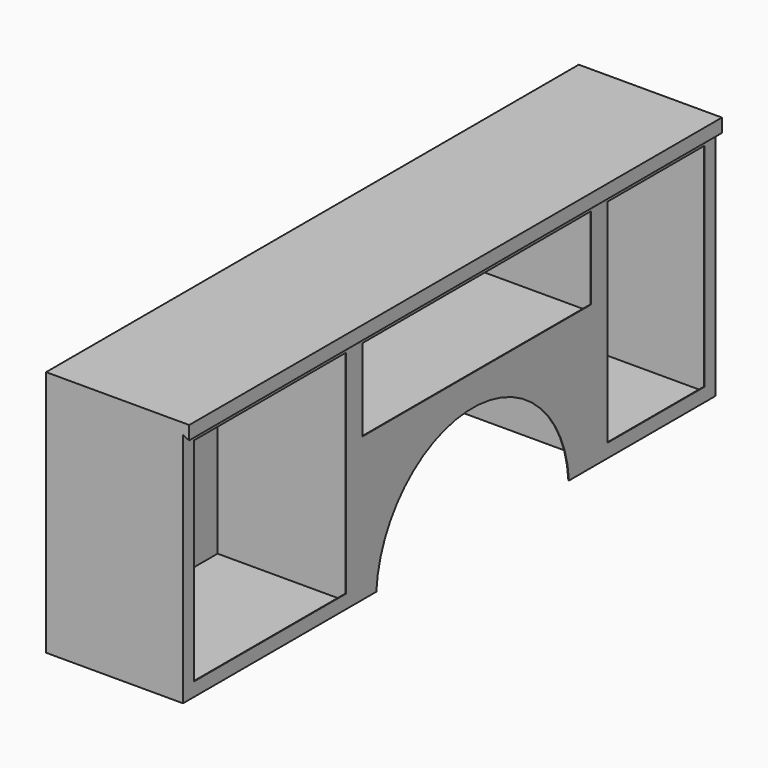
from build123d import *

# Parameters (mm, degrees)
F0_W      = 508
F0_H      = 914.4
F1_DEPTH  = 2470.15
F2_W      = 704.85
F2_H      = 787.4
F2_W_2    = 1060.45
F2_H_2    = 304.8
F2_W_3    = 450.85
F3_DEPTH  = 505.8918
F4_W      = 503.7836
F4_H      = 704.85
F5_DEPTH  = 48.6918
F6_W      = 503.7836
F6_H      = 704.85
F7_DEPTH  = 48.6918
F8_W      = 503.7836
F8_H      = 884.7836
F9_DEPTH  = 48.6918
F10_W     = 503.7836
F10_H     = 884.7836
F11_DEPTH = 37.0459
F12_W     = 503.7836
F12_H     = 1060.45
F13_DEPTH = 48.6918
F14_W     = 503.7836
F14_H     = 1060.45
F15_DEPTH = 48.6918
F16_W     = 503.7836
F16_H     = 402.1836
F17_DEPTH = 37.0459
F18_W     = 503.7836
F18_H     = 402.1836
F19_DEPTH = 37.0459
F20_W     = 503.7836
F20_H     = 450.85
F21_DEPTH = 48.6918
F22_W     = 503.7836
F22_H     = 450.85
F23_DEPTH = 48.6918
F24_W     = 503.7836
F24_H     = 884.7836
F25_DEPTH = 37.0459
F26_W     = 503.7836
F26_H     = 884.7836
F27_DEPTH = 48.6918
F28_W     = 505.8918
F28_H     = 1134.5418
F29_DEPTH = 482.6
F31_DEPTH = 508.001
F33_DEPTH = 2470.15
F34_R     = 0.508


with BuildPart() as f1:
    # F0 (on Front) → F1 (new body)
    with BuildSketch(Plane.XZ):
        Rectangle(F0_W, F0_H)
    extrude(amount=-F1_DEPTH)

    # F2 (on face) → F3 (cut)
    with BuildSketch(Plane.YZ.offset(254)):
        with Locations((403.225, -12.7)):
            Rectangle(F2_W, F2_H)
        with Locations((1362.075, 228.6)):
            Rectangle(F2_W_2, F2_H_2)
        with Locations((2193.925, -12.7)):
            Rectangle(F2_W_3, F2_H)
    extrude(amount=-F3_DEPTH, mode=Mode.SUBTRACT)

    # F4 (on face) → F5 (cut)
    with BuildSketch(Plane.XY.offset(-406.4)):
        with Locations((0, 403.225)):
            Rectangle(F4_W, F4_H)
    extrude(amount=-F5_DEPTH, mode=Mode.SUBTRACT)

    # F6 (on face) → F7 (cut)
    with BuildSketch(Plane(origin=(0, 0, 381), x_dir=(1, 0, 0), z_dir=(0, 0, -1))):
        with Locations((0, -403.225)):
            Rectangle(F6_W, F6_H)
    extrude(amount=-F7_DEPTH, mode=Mode.SUBTRACT)

    # F8 (on face) → F9 (cut)
    with BuildSketch(Plane(origin=(0, 50.8, 0), x_dir=(-1, 0, 0), z_dir=(0, 1, 0))):
        with Locations((0, -12.7)):
            Rectangle(F8_W, F8_H)
    extrude(amount=-F9_DEPTH, mode=Mode.SUBTRACT)

    # F10 (on face) → F11 (cut)
    with BuildSketch(Plane.XZ.offset(-755.65)):
        with Locations((0, -12.7)):
            Rectangle(F10_W, F10_H)
    extrude(amount=-F11_DEPTH, mode=Mode.SUBTRACT)

    # F12 (on face) → F13 (cut)
    with BuildSketch(Plane.XY.offset(76.2)):
        with Locations((0, 1362.075)):
            Rectangle(F12_W, F12_H)
    extrude(amount=-F13_DEPTH, mode=Mode.SUBTRACT)

    # F14 (on face) → F15 (cut)
    with BuildSketch(Plane(origin=(0, 0, 381), x_dir=(1, 0, 0), z_dir=(0, 0, -1))):
        with Locations((0, -1362.075)):
            Rectangle(F14_W, F14_H)
    extrude(amount=-F15_DEPTH, mode=Mode.SUBTRACT)

    # F16 (on face) → F17 (cut)
    with BuildSketch(Plane(origin=(0, 831.85, 0), x_dir=(-1, 0, 0), z_dir=(0, 1, 0))):
        with Locations((0, 228.6)):
            Rectangle(F16_W, F16_H)
    extrude(amount=-F17_DEPTH, mode=Mode.SUBTRACT)

    # F18 (on face) → F19 (cut)
    with BuildSketch(Plane.XZ.offset(-1892.3)):
        with Locations((0, 228.6)):
            Rectangle(F18_W, F18_H)
    extrude(amount=-F19_DEPTH, mode=Mode.SUBTRACT)

    # F20 (on face) → F21 (cut)
    with BuildSketch(Plane.XY.offset(-406.4)):
        with Locations((0, 2193.925)):
            Rectangle(F20_W, F20_H)
    extrude(amount=-F21_DEPTH, mode=Mode.SUBTRACT)

    # F22 (on face) → F23 (cut)
    with BuildSketch(Plane(origin=(0, 0, 381), x_dir=(1, 0, 0), z_dir=(0, 0, -1))):
        with Locations((0, -2193.925)):
            Rectangle(F22_W, F22_H)
    extrude(amount=-F23_DEPTH, mode=Mode.SUBTRACT)

    # F24 (on face) → F25 (cut)
    with BuildSketch(Plane(origin=(0, 1968.5, 0), x_dir=(-1, 0, 0), z_dir=(0, 1, 0))):
        with Locations((0, -12.7)):
            Rectangle(F24_W, F24_H)
    extrude(amount=-F25_DEPTH, mode=Mode.SUBTRACT)

    # F26 (on face) → F27 (cut)
    with BuildSketch(Plane.XZ.offset(-2419.35)):
        with Locations((0, -12.7)):
            Rectangle(F26_W, F26_H)
    extrude(amount=-F27_DEPTH, mode=Mode.SUBTRACT)

    # F28 (on face) → F29 (cut)
    with BuildSketch(Plane(origin=(0, 0, -457.2), x_dir=(1, 0, 0), z_dir=(0, 0, -1))):
        with Locations((-1.0541, -1362.075)):
            Rectangle(F28_W, F28_H)
    extrude(amount=-F29_DEPTH, mode=Mode.SUBTRACT)

    # F30 (on face) → F31 (cut, through all)
    with BuildSketch(Plane.YZ.offset(254)):
        with BuildLine():
            Line((896.4041, -457.2), (1789.6459, -457.2))
            ThreePointArc((1789.6459, -457.2), (1343.025, -38.1), (896.4041, -457.2))
        make_face()
    extrude(amount=-F31_DEPTH, mode=Mode.SUBTRACT)

    # F32 (on face) → F33 (join, through all)
    with BuildSketch(Plane.XZ):
        Polygon((277.0862247403, 459.3082), (-254, 459.3082), (-254, 457.2), (254, 457.2), (254, 419.1), (277.0862247403, 408.5082), align=None)
    extrude(amount=-F33_DEPTH)

    # F34
    f34_edges = [f1.edges().sort_by_distance(p)[0] for p in [
        (277.086225, 1235.075, 408.5082),
    ]]
    fillet(f34_edges, radius=F34_R)


solid = f1.part
